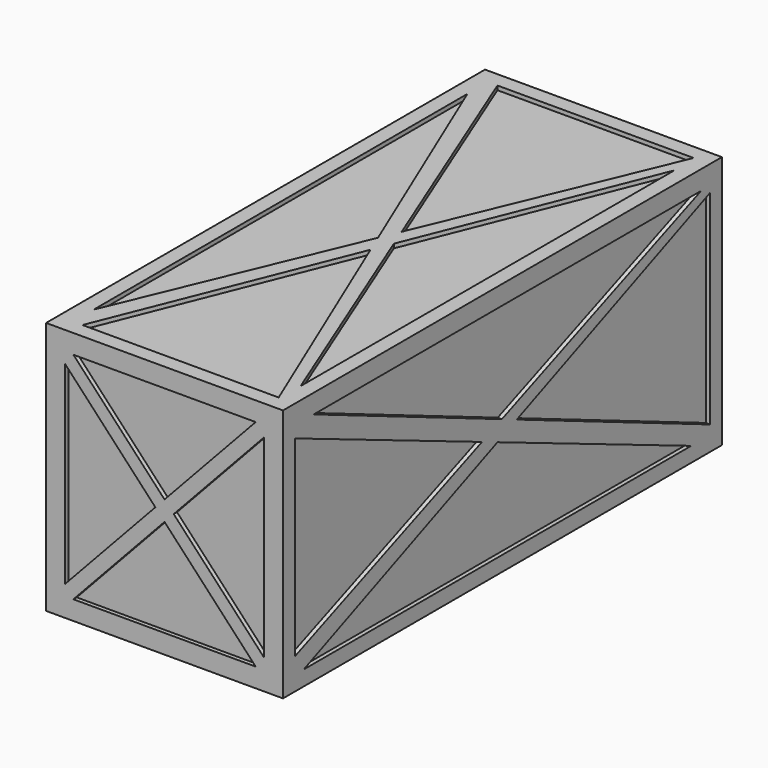
from build123d import *

# Parameters (mm, degrees)
F0_W     = 27.5
F0_H     = 66
F1_DEPTH = 30
F2_W     = 66
F2_H     = 30
F3_DEPTH = 0.5
F4_W     = 28.5
F4_H     = 66
F5_DEPTH = 0.5
F7_DEPTH = 0.5
F8_W     = 20.5
F8_H     = 58
F9_DEPTH = 28.5
F10_R    = 10.24999


# Not quite as in the source:
# - two fillets or chamfers of one size are made in one step
# - a fillet or chamfer is up to 0.001 mm smaller than in the source, because OpenCascade refuses the exact size
# - a pattern or mirror of a feature is missing from the dataset's text; its kind, count and spacing are read off the source's solid


with BuildPart() as f1:
    # F0 (on Top) → F1 (new body)
    with BuildSketch(Plane.XY):
        Rectangle(F0_W, F0_H)
    extrude(amount=F1_DEPTH)

    # F2 (on face) → F3 (join)
    with BuildSketch(Plane.YZ.offset(13.75)):
        with Locations((0, 15)):
            Rectangle(F2_W, F2_H)
        Polygon((28.3744677029, 1.8), (-29.8744677029, 1.8), (-0.75, 14.0239419294), align=None, mode=Mode.SUBTRACT)
        Polygon((-31.2, 3.7331419218), (-31.2, 26.8042280979), (-3.0755322971, 15), align=None, mode=Mode.SUBTRACT)
        Polygon((-0.0901844103, 16.195951202), (-28.3744677029, 28.2), (29.8744677029, 28.2), align=None, mode=Mode.SUBTRACT)
        Polygon((31.2, 27.4337988451), (31.2, 2.9161768244), (2.1548442575, 15.2431452425), align=None, mode=Mode.SUBTRACT)
    f3 = extrude(amount=F3_DEPTH)

    # F3_copies: F3 across plane
    add(f3.mirror(Plane(origin=(0, 0, 0), x_dir=(0, 0, -1), z_dir=(-1, 0, 0))))

    # F4 (on face) → F5 (join)
    with BuildSketch(Plane.XY.offset(30)):
        Rectangle(F4_W, F4_H)
        Polygon((0.25, -2.338037696), (12.2876657229, -31.2), (-11.3137418755, -31.2), align=None, mode=Mode.SUBTRACT)
        Polygon((-0.7251421589, 0), (-12.45, -28.111962304), (-12.45, 28.111962304), align=None, mode=Mode.SUBTRACT)
        Polygon((1.1867507353, 0), (12.45, 28.111962304), (12.45, -28.111962304), align=None, mode=Mode.SUBTRACT)
        Polygon((0.25, 2.338037696), (-11.3137418755, 31.2), (12.2876657229, 31.2), align=None, mode=Mode.SUBTRACT)
    extrude(amount=F5_DEPTH)

    # F6 (on face) → F7 (cut)
    with BuildSketch(Plane.XZ.offset(33)):
        Polygon((0, 14.0644738981), (-10.9635152767, 2.3), (10.9635152767, 2.3), align=None)
        Polygon((-1.1048121354, 15.25), (-11.95, 26.8875018716), (-11.95, 3.6124981284), align=None)
        Polygon((0, 16.4355261019), (10.9635152767, 28.2), (-10.9635152767, 28.2), align=None)
        Polygon((1.1048121354, 15.25), (11.95, 3.6124981284), (11.95, 26.8875018716), align=None)
    f7 = extrude(amount=-F7_DEPTH, mode=Mode.SUBTRACT)

    # F7_copies: F7 across plane
    add(f7.mirror(Plane.ZX), mode=Mode.SUBTRACT)

    # F8 (on face) → F9 (cut)
    with BuildSketch(Plane(origin=(0, 0, 0), x_dir=(1, 0, 0), z_dir=(0, 0, -1))):
        Rectangle(F8_W, F8_H)
    extrude(amount=-F9_DEPTH, mode=Mode.SUBTRACT)

    # F10 (radius 10.25 in the source; OpenCascade refuses exactly that, so slightly less here)
    f10_edges = [f1.edges().sort_by_distance(p)[0] for p in [
        (-10.25, 0, 28.5),
        (10.25, 0, 28.5),
    ]]
    fillet(f10_edges, radius=F10_R)


solid = f1.part
